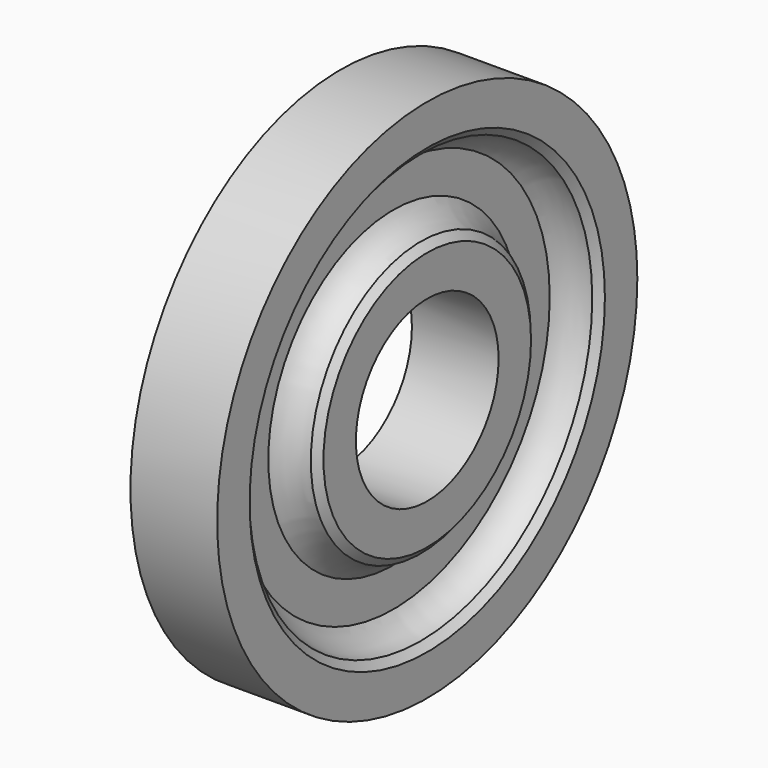
from build123d import *

# Parameters (mm, degrees)
F4_D     = 16
F4_DEPTH = 302.871


# Not quite as in the source:
# - a fillet or chamfer that OpenCascade refuses, or shapes differently, is made with other operations: its cross-section is extruded or revolved along the edge and cut away or added


with BuildPart() as f1:
    # F0 (on Top) → F1 (revolve)
    with BuildSketch(Plane.XY):
        with BuildLine():
            Line((0, 302.87), (-100, 302.87))
            Line((-100, 302.87), (-100, 240.87))
            ThreePointArc((-100, 240.87), (-113.9805777598, 238.2047342639), (-126, 230.5828129211))
            Line((-126, 230.5828129211), (-126, 175.1571870789))
            ThreePointArc((-126, 175.1571870789), (-113.9805777598, 167.5352657361), (-100, 164.87))
            Line((-100, 164.87), (-100, 102.87))
            Line((-100, 102.87), (0, 102.87))
            Line((0, 102.87), (0, 157.87))
            ThreePointArc((0, 157.87), (-22.5250139353, 163.9133093395), (-39, 180.4200556794))
            Line((-39, 180.4200556794), (-39, 225.3199443206))
            ThreePointArc((-39, 225.3199443206), (-22.5250139353, 241.8266906605), (0, 247.87))
            Line((0, 247.87), (0, 302.87))
        make_face()
    revolve(axis=Axis((-229.3646931648, 0, 0), (1, 0, 0)))

    # F2: chamfer of 9 on 2 edges, made by hand

    # F2_s1 → F2_t2 (revolve, cut)
    with BuildSketch(Plane.XY):
        with BuildLine():
            Line((-7.5, 247.2405983732), (0, 256.1147180479))
            Line((0, 256.1147180479), (0, 247.87))
            ThreePointArc((0, 247.87), (-3.8908074648, 247.7014802039), (-7.5, 247.2405983732))
        make_face()
    revolve(axis=Axis((0, 0, 0), (1, 0, 0)), mode=Mode.SUBTRACT)

    # F2_s3 → F2_t4 (revolve, cut)
    with BuildSketch(Plane.XY):
        with BuildLine():
            Line((0, 149.6252819521), (-7.5, 158.4994016268))
            ThreePointArc((-7.5, 158.4994016268), (-3.8908074648, 158.0385197961), (0, 157.87))
            Line((0, 157.87), (0, 149.6252819521))
        make_face()
    revolve(axis=Axis((0, 0, 0), (1, 0, 0)), mode=Mode.SUBTRACT)

    # F4 (through all, one way)
    with BuildSketch(Plane.XY):
        with Locations((-77.5457248092, 302.87)):
            Circle(F4_D / 2)
    extrude(amount=-F4_DEPTH, mode=Mode.SUBTRACT)


solid = f1.part
